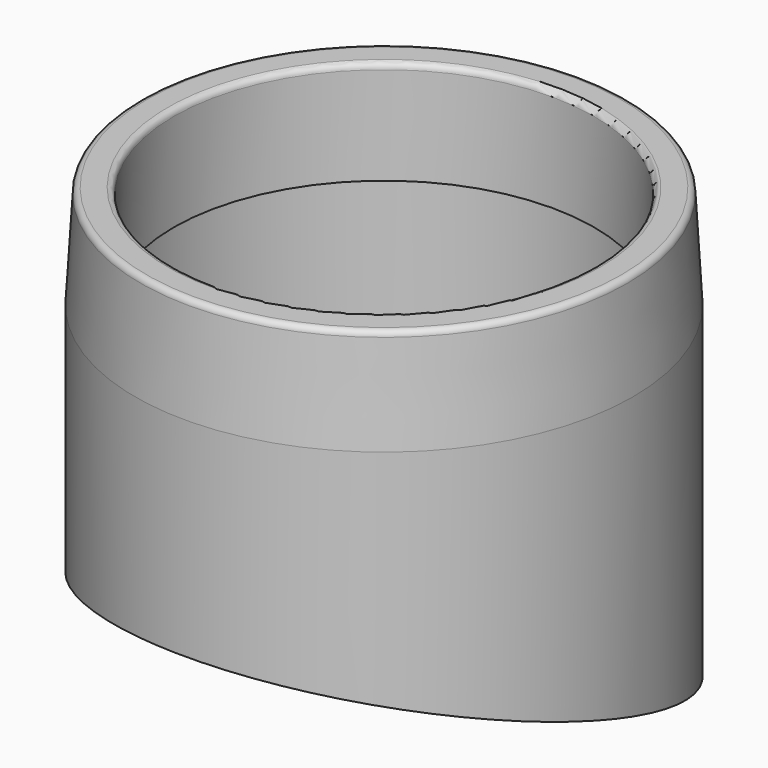
from build123d import *

# Parameters (mm, degrees)
F0_R     = 42
F0_R_2   = 35.5
F1_DEPTH = 17.5
F2_SIZE2 = 17.49999
F2_SIZE  = 0.99999
F3_R     = 1
F4_R     = 42
F4_R_2   = 37
F5_DEPTH = 60
F7_DEPTH = 45


# Not quite as in the source:
# - a fillet or chamfer is up to 0.001 mm smaller than in the source, because OpenCascade refuses the exact size


with BuildPart() as f1:
    # F0 (on Top) → F1 (new body)
    with BuildSketch(Plane.XY):
        Circle(F0_R)
        Circle(F0_R_2, mode=Mode.SUBTRACT)
    extrude(amount=F1_DEPTH)

    # F2 (size 1 and 17.5 in the source; OpenCascade refuses exactly that, so slightly less here)
    f2_edges = [f1.edges().sort_by_distance(p)[0] for p in [
        (-42, 0, 17.5),
    ]]
    f2_side = f1.faces().sort_by_distance((-40.812061, 0, 17.5))[0]
    chamfer(f2_edges, length=F2_SIZE, length2=F2_SIZE2, reference=f2_side)

    # F3
    f3_edges = [f1.edges().sort_by_distance(p)[0] for p in [
        (-41.00001, 0, 17.5),
        (-35.5, 0, 17.5),
    ]]
    fillet(f3_edges, radius=F3_R)


with BuildPart() as f5:
    # F4 (on face) → F5 (new body)
    with BuildSketch(Plane(origin=(0, 0, 0), x_dir=(1, 0, 0), z_dir=(0, 0, -1))):
        Circle(F4_R)
        Circle(F4_R_2, mode=Mode.SUBTRACT)
    extrude(amount=F5_DEPTH)

    # F6 (on Right) → F7 (cut, symmetric)
    with BuildSketch(Plane.YZ):
        Polygon((42.5, -69.3717226386), (42.5, -60), (-42.5, -35), (-49.787659198, -69.3717226386), align=None)
    extrude(amount=F7_DEPTH, both=True, mode=Mode.SUBTRACT)


solid = Compound([f1.part, f5.part])
